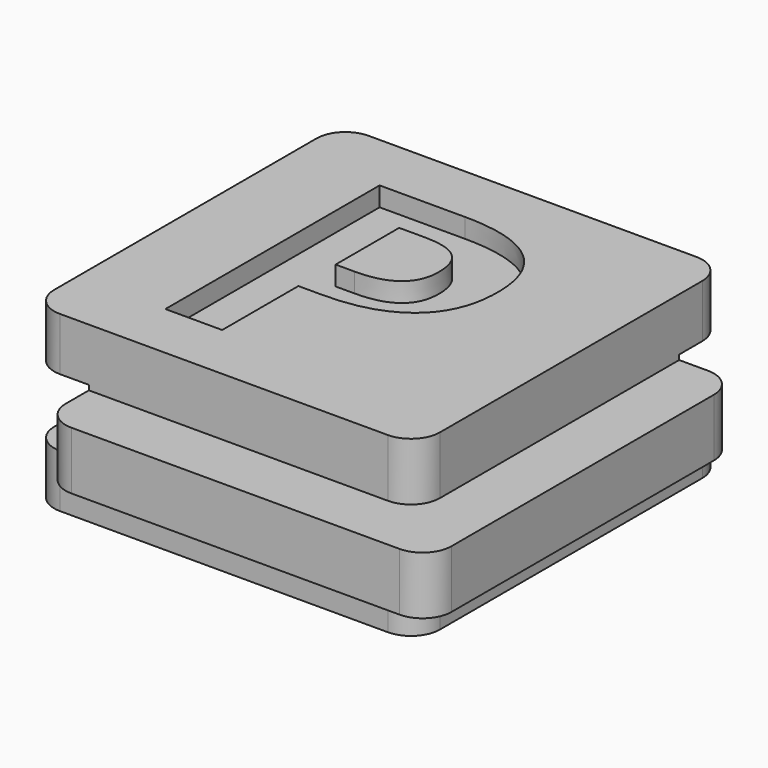
from build123d import *

# Parameters (mm, degrees)
F0_W         = 14
F0_H         = 3
F0_W_2       = 3
F1_DEPTH     = 20
F2_DEPTH     = 3
F3_W         = 3
F3_H         = 3
F4_DEPTH     = 100
F5_W         = 3
F5_H         = 3.5
F6_DEPTH     = 100
F7_R         = 1.5
F8_TEXT_SIZE = 19.4444444444
F9_DEPTH     = 1


# Not quite as in the source:
# - Text() gives the source's letters only with a copy of the font that has no kerning and outlines rounded to 1/6400 em; it was checked with that copy


with BuildPart() as f1:
    # F0 (on Front) → F1 (new body)
    with BuildSketch(Plane.XZ):
        Polygon((10, 1.5), (10, 4.5), (-10, 4.5), (-10, 1.5), (-7, 1.5), (7, 1.5), align=None)
        Rectangle(F0_W, F0_H)
        with Locations((11.5, 0)):
            Rectangle(F0_W_2, F0_H)
        with Locations((8.5, 0)):
            Rectangle(F0_W_2, F0_H)
        with Locations((-8.5, 0)):
            Rectangle(F0_W_2, F0_H)
        Polygon((10, -4.5), (10, -1.5), (7, -1.5), (-7, -1.5), (-10, -1.5), (-10, -4.5), align=None)
    extrude(amount=-F1_DEPTH)

    # F0 (on Front) → F2 (join)
    with BuildSketch(Plane.XZ):
        with Locations((-8.5, 0)):
            Rectangle(F0_W_2, F0_H)
        Rectangle(F0_W, F0_H)
        with Locations((8.5, 0)):
            Rectangle(F0_W_2, F0_H)
        with Locations((11.5, 0)):
            Rectangle(F0_W_2, F0_H)
    extrude(amount=F2_DEPTH)

    # F3 (on face) → F4 (cut)
    with BuildSketch(Plane.YZ.offset(13)):
        Polygon((23, -1.75), (23, 1.75), (17, 1.75), (17, 1.5), (20, 1.5), (20, -1.5), (17, -1.5), (17, -1.75), align=None)
        with Locations((18.5, 0)):
            Rectangle(F3_W, F3_H)
    extrude(amount=-F4_DEPTH, mode=Mode.SUBTRACT)

    # F5 (on face) → F6 (cut)
    with BuildSketch(Plane(origin=(0, 17, 0), x_dir=(-1, 0, 0), z_dir=(0, 1, 0))):
        with Locations((11.5, 0)):
            Rectangle(F5_W, F5_H)
        with Locations((8.5, 0)):
            Rectangle(F5_W, F5_H)
    extrude(amount=-F6_DEPTH, mode=Mode.SUBTRACT)

    # F7
    f7_edges = [f1.edges().sort_by_distance(p)[0] for p in [
        (-7, -3, 0),
        (13, -3, 0),
        (10, 0, 3),
        (10, 0, -3),
        (-10, 0, -3.125),
        (-10, 0, 3.125),
        (-7, 17, 0),
        (-10, 20, 3.125),
        (-10, 20, -3.125),
        (13, 17, 0),
        (10, 20, 3.125),
        (10, 20, -3.125),
    ]]
    fillet(f7_edges, radius=F7_R)

    # F8 (on face) → F9 (cut)
    with BuildSketch(Plane.XY.offset(4.5)):
        with Locations((-7.1801951318, 3)):
            Text('P', F8_TEXT_SIZE, font='Open Sans', font_style=FontStyle.BOLD, text_align=(TextAlign.LEFT, TextAlign.BOTTOM))
    extrude(amount=-F9_DEPTH, mode=Mode.SUBTRACT)


solid = f1.part
